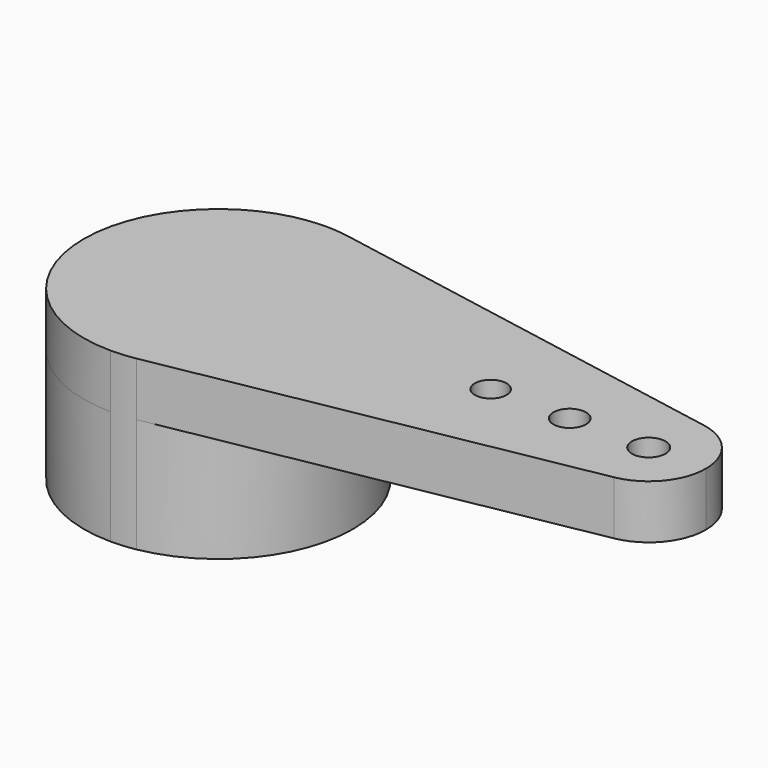
from build123d import *

# Parameters (mm, degrees)
F0_W     = 4
F0_H     = 3.4
F2_DEPTH = 4
F4_DEPTH = 25
F3_R     = 0.471746
F3_R_2   = 0.5
F3_R_3   = 0.485204
F5_DEPTH = 25


# Not quite as in the source:
# - after a boolean that leaves OpenCascade's solid faulty, fix() repairs it


with BuildPart() as f1:
    # F0 (on Front) → F1 (revolve)
    with BuildSketch(Plane.XZ):
        with Locations((2, 1.7)):
            Rectangle(F0_W, F0_H)
    revolve(axis=Axis((0, 0, 1.7), (0, 0, 1)))

    # F0 (on Front) → F2 (join, symmetric)
    with BuildSketch(Plane.XZ):
        Polygon((-4, 3.4), (0, 3.4), (4, 3.4), (14.5, 3.4), (14.5, 5), (-4, 5), align=None)
    extrude(amount=F2_DEPTH, both=True)

    # F3 (on face) → F4 (cut)
    with BuildSketch(Plane.XY.offset(5)):
        with BuildLine():
            Line((13.105469, -1.67233), (0.71875, -3.934895))
            ThreePointArc((0.71875, -3.934895), (0.360846, -3.98369), (0, -4))
            Line((0, -4), (14.5, -4))
            Line((14.5, -4), (14.5, 0))
            ThreePointArc((14.5, 0), (14.105622, -1.088739), (13.105469, -1.67233))
        make_face()
        with BuildLine():
            ThreePointArc((0, 4), (0.360846, 3.98369), (0.71875, 3.934895))
            Line((0.71875, 3.934895), (13.105469, 1.67233))
            ThreePointArc((13.105469, 1.67233), (14.105622, 1.088739), (14.5, 0))
            Line((14.5, 0), (14.5, 4))
            Line((14.5, 4), (0, 4))
        make_face()
        with BuildLine():
            ThreePointArc((-4, 0), (-2.828427, 2.828427), (0, 4))
            Line((0, 4), (-4, 4))
            Line((-4, 4), (-4, 0))
        make_face()
        with BuildLine():
            Line((-4, -4), (0, -4))
            ThreePointArc((0, -4), (-2.828427, -2.828427), (-4, 0))
            Line((-4, 0), (-4, -4))
        make_face()
    extrude(amount=-F4_DEPTH, mode=Mode.SUBTRACT)

    add(f1.part.fix(), mode=Mode.REPLACE)

    # F3 (on face) → F5 (cut)
    with BuildSketch(Plane.XY.offset(5)):
        with Locations((8.1, 0)):
            Circle(F3_R)
        with Locations((12.8, 0)):
            Circle(F3_R_2)
        with Locations((10.45, 0)):
            Circle(F3_R_3)
    extrude(amount=-F5_DEPTH, mode=Mode.SUBTRACT)


solid = f1.part
